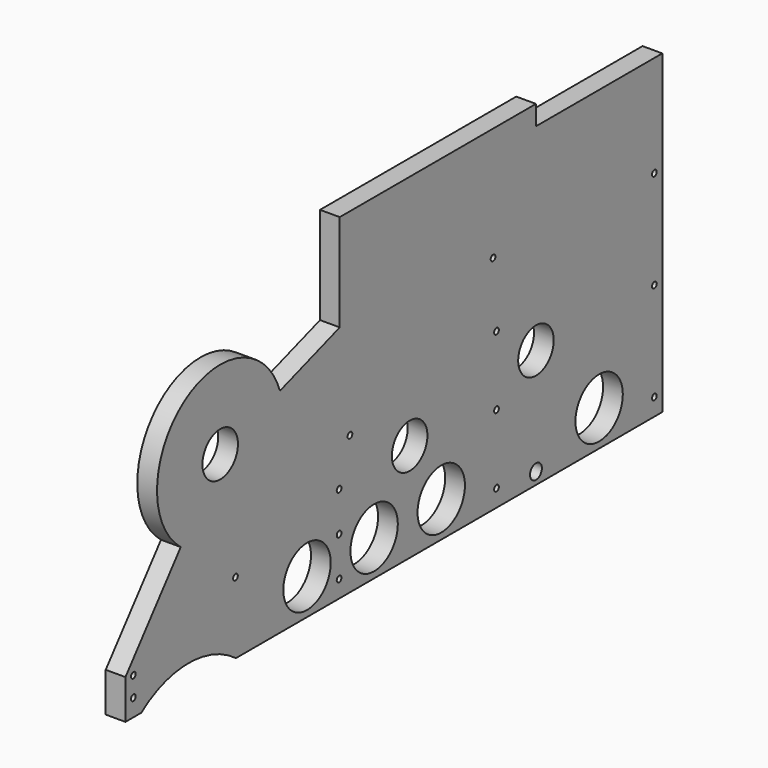
from build123d import *

# Parameters (mm, degrees)
F0_R     = 1.905
F0_R_2   = 14.2875
F0_R_3   = 4.7625
F1_DEPTH = 12.7
F2_R     = 19.05
F3_DEPTH = 12.7
F5_DEPTH = 12.7
F6_R     = 1.905
F7_DEPTH = 12.7


with BuildPart() as f1:
    # F0 (on Right) → F1 (new body)
    with BuildSketch(Plane.YZ):
        with BuildLine():
            Line((0, 355.6), (0, 0))
            Line((0, 0), (12.7, 0))
            ThreePointArc((12.7, 0), (50.8, 12.7), (88.9, 0))
            Line((88.9, 0), (431.8, 0))
            Line((431.8, 0), (431.8, 355.6))
            Line((431.8, 355.6), (0, 355.6))
        make_face()
        with Locations((88.4877131973, 46.0377095938)):
            Circle(F0_R, mode=Mode.SUBTRACT)
        with Locations((180.5685843602, 88.9757249866)):
            Circle(F0_R, mode=Mode.SUBTRACT)
        with Locations((228.6, 63.5)):
            Circle(F0_R_2, mode=Mode.SUBTRACT)
        with Locations((330.2, 7.62)):
            Circle(F0_R_3, mode=Mode.SUBTRACT)
        with Locations((330.2, 76.2)):
            Circle(F0_R_2, mode=Mode.SUBTRACT)
        with Locations((76.2, 120.65)):
            Circle(F0_R_2, mode=Mode.SUBTRACT)
        with Locations((295.6696733139, 142.6482442277)):
            Circle(F0_R, mode=Mode.SUBTRACT)
    extrude(amount=F1_DEPTH)

    # F2 (on face) → F3 (cut, through all)
    with BuildSketch(Plane.YZ.offset(12.7)):
        with Locations((146.05, 23.05)):
            Circle(F2_R)
        with Locations((254, 23.05)):
            Circle(F2_R)
        with Locations((381, 23.0378)):
            Circle(F2_R)
        with Locations((200.025, 23.05)):
            Circle(F2_R)
    extrude(amount=-F3_DEPTH, mode=Mode.SUBTRACT)

    # F4 (on face) → F5 (cut, through all)
    with BuildSketch(Plane.YZ.offset(12.7)):
        Polygon((431.8, 355.6), (0, 355.6), (0, 215.9), (172.3654351189, 215.9), (330.2, 215.9), (355.6, 215.9), (431.8, 215.9), align=None)
        with BuildLine():
            Line((172.3654351189, 215.9), (0, 215.9))
            Line((0, 215.9), (0, 25.4))
            Line((0, 25.4), (44.4654915842, 80.9818644803))
            ThreePointArc((44.4654915842, 80.9818644803), (47.0024645882, 162.2209505049), (124.2827175595, 137.0418355316))
            Line((124.2827175595, 137.0418355316), (172.3654351189, 153.4336710633))
            Line((172.3654351189, 153.4336710633), (172.3654351189, 215.9))
        make_face()
        Polygon((431.8, 203.2), (431.8, 215.9), (355.6, 215.9), (330.2, 207.2409090909), (330.2, 203.2), align=None)
        Polygon((330.2, 207.2409090909), (355.6, 215.9), (330.2, 215.9), align=None)
    extrude(amount=-F5_DEPTH, mode=Mode.SUBTRACT)

    # F6 (on face) → F7 (cut, through all)
    with BuildSketch(Plane.YZ.offset(12.7)):
        with Locations((425.45, 11.1125)):
            Circle(F6_R)
        with Locations((425.45, 74.5109)):
            Circle(F6_R)
        with Locations((425.45, 137.9093)):
            Circle(F6_R)
        with Locations((298.45, 11.1125)):
            Circle(F6_R)
        with Locations((298.45, 100.0125)):
            Circle(F6_R)
        with Locations((298.45, 55.5625)):
            Circle(F6_R)
        with Locations((171.8554794788, 11.1125)):
            Circle(F6_R)
        with Locations((171.8554794788, 36.5125)):
            Circle(F6_R)
        with Locations((171.8554794788, 61.9125)):
            Circle(F6_R)
        with Locations((6.35, 11.1125)):
            Circle(F6_R)
        with Locations((6.35, 23.8125)):
            Circle(F6_R)
    extrude(amount=-F7_DEPTH, mode=Mode.SUBTRACT)


solid = f1.part
